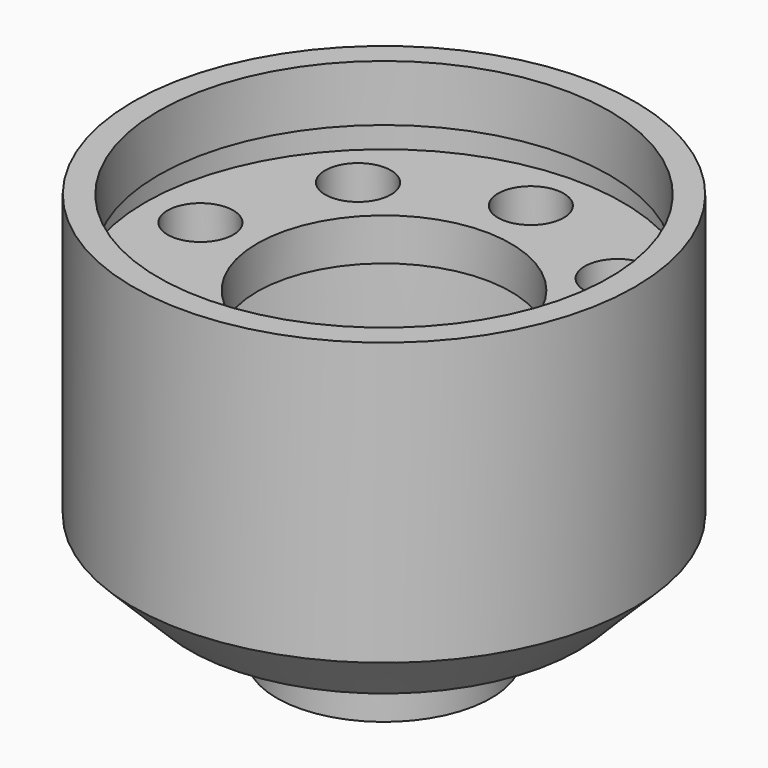
from build123d import *

# Parameters (mm, degrees)
F0_W     = 2.5722222222
F0_H     = 10.2888888889
F2_R     = 6
F3_DEPTH = 12.5


# Not quite as in the source:
# - ends of sketch curves that miss each other by under 0.0002 mm in the source are joined
# - a feature names something its author has since deleted; it is built from what else it names


with BuildPart() as f1:
    # F0 (on Front) → F1 (revolve)
    with BuildSketch(Plane.XZ):
        Polygon((-42.2873333333, 14.7902777778), (-43.4808444444, 14.7902777778), (-43.7277777778, 14.7902777778), (-43.7277777778, 25.0791666667), (-43.7277777778, 27.6513888889), (-43.7277777778, 37.9402777778), (-45.7855555556, 37.9402777778), (-45.7855555556, -13.5041666667), (-35.4966666667, -23.7930555556), (-23.15, -23.7930555556), (-19.5720388889, -23.7930555556), (-19.5488888889, -23.7930555556), (-19.5488888889, -36.6541666667), (-17.1001333333, -36.6541666667), (-17.1001333333, -35.0491), (-17.1307942222, -33.3098044889), (-16.0422915111, -33.2906054222), (-16.0422915111, -33.2845967111), (-16.0422915111, -33.278588), (-16.0422915111, -33.2725792889), (-16.0422915111, -33.2665705778), (-16.0422915111, -33.2605618667), (-16.0422915111, -33.2545531556), (-16.0422915111, -33.2485444444), (-16.0422915111, -33.2425357333), (-16.0422915111, -33.2365270222), (-16.0422915111, -33.2305183111), (-16.0422915111, -33.2245096), (-16.0422915111, -33.2185008889), (-16.0422915111, -33.2124921778), (-16.0422915111, -33.2064834667), (-16.0422915111, -33.2004747556), (-16.0422915111, -33.1944660444), (-16.0422915111, -33.1884573333), (-16.0422915111, -33.1824486222), (-16.0422915111, -33.1764604889), (-16.0422915111, -33.1704517778), (-16.0422915111, -33.1644430667), (-16.0422915111, -33.1584343556), (-16.0422915111, -33.1524256444), (-16.0422915111, -33.1464169333), (-16.0426824889, -33.1284731111), (-16.0438554222, -33.1105292889), (-16.0458103111, -33.0926677778), (-16.0485471556, -33.074868), (-16.0520659556, -33.0572534222), (-16.0563255556, -33.0398240444), (-16.0613465333, -33.0226004444), (-16.0671288889, -33.0056032), (-16.0736314667, -32.9888734667), (-16.0808748444, -32.9724112444), (-16.0888384444, -32.9562782667), (-16.0975016889, -32.9405156889), (-16.1068028444, -32.9251646667), (-16.1167830667, -32.9102663556), (-16.1273806222, -32.8958207556), (-16.1385955111, -32.8818484444), (-16.1504071556, -32.86837), (-16.1628361333, -32.855406), (-16.1758001333, -32.8429770222), (-16.1893403111, -32.8311036444), (-16.2033537778, -32.8198681778), (-16.2178405333, -32.8092500444), (-16.2327388444, -32.7992904), (-16.2480692889, -32.7899892444), (-16.2772074222, -32.7731772), (-16.3063455556, -32.7563445778), (-16.3354836889, -32.7395119556), (-16.3646218222, -32.7226999111), (-16.3937599556, -32.7058672889), (-16.4229186667, -32.6890552444), (-16.4520568, -32.6722226222), (-16.4811949333, -32.65539), (-16.5103330667, -32.6385779556), (-16.5394712, -32.6217453333), (-16.5686093333, -32.6049127111), (-16.5977474667, -32.5881006667), (-16.6268856, -32.5712680444), (-16.6560443111, -32.554456), (-16.6851824444, -32.5376233778), (-16.7143205778, -32.5207907556), (-16.7434587111, -32.5039787111), (-16.7725968444, -32.4871460889), (-16.8017349778, -32.4703340444), (-16.8308731111, -32.4535014222), (-16.8600318222, -32.4366688), (-16.8891699556, -32.4198567556), (-16.9183080889, -32.4030241333), (-16.9474462222, -32.3862120889), (-16.9625708889, -32.3770344), (-16.977284, -32.3672188), (-16.9915444, -32.3568064444), (-17.0053315111, -32.3457973333), (-17.0186453333, -32.3341914667), (-17.0314447111, -32.32203), (-17.0437296444, -32.3093129333), (-17.0554795556, -32.2960608444), (-17.0666327111, -32.2823354667), (-17.0771685333, -32.2681573778), (-17.0870870222, -32.2535471556), (-17.0963676, -32.2385253778), (-17.1049896889, -32.2231332), (-17.1129532889, -32.2073500444), (-17.1202584, -32.1912376444), (-17.1268432889, -32.1748165778), (-17.1327285333, -32.1581485778), (-17.1378729778, -32.1412748), (-17.1422766222, -32.1242158222), (-17.1459600444, -32.1069716444), (-17.1489026667, -32.089604), (-17.1511044889, -32.0720923111), (-17.1525449333, -32.0544777333), (-17.1532445778, -32.0368014222), (-17.1690071556, -31.1425529333), (-17.1689248444, -31.1242387111), (-17.16804, -31.1059862222), (-17.1663320444, -31.0878160444), (-17.1638215556, -31.0697281778), (-17.1605291111, -31.0517843556), (-17.1564341333, -31.0339845778), (-17.1515366222, -31.0163494222), (-17.1458571556, -30.9989406222), (-17.1394368889, -30.9818199111), (-17.1322552444, -30.9650284444), (-17.1243328, -30.9485662222), (-17.1157107111, -30.9324949778), (-17.1063684, -30.9167941333), (-17.0963264444, -30.9015254222), (-17.085626, -30.8867094222), (-17.0742464889, -30.8723461333), (-17.0622702222, -30.8585590222), (-17.0497177778, -30.8453069333), (-17.0365891556, -30.8326516), (-17.0229255111, -30.8205724444), (-17.0087268444, -30.8091312), (-16.9940343111, -30.7983072889), (-16.9788684889, -30.7881418667), (-16.9632293778, -30.7786349333), (-16.9359432444, -30.7628929333), (-16.9086571111, -30.7471303556), (-16.8813915556, -30.7313883556), (-16.8541054222, -30.7156463556), (-16.8268192889, -30.6998837778), (-16.7995537333, -30.6841417778), (-16.7722676, -30.6683997778), (-16.7449814667, -30.6526372), (-16.7177159111, -30.6368952), (-16.6904297778, -30.6211532), (-16.6631436444, -30.6053906222), (-16.6358780889, -30.5896486222), (-16.6085919556, -30.5738860444), (-16.5813058222, -30.5581440444), (-16.5540402667, -30.5424020444), (-16.5267541333, -30.5266394667), (-16.4994885778, -30.5108974667), (-16.4722024444, -30.4951554667), (-16.4449163111, -30.4793928889), (-16.4176507556, -30.4636508889), (-16.3903646222, -30.4478883111), (-16.3630784889, -30.4321463111), (-16.3358129333, -30.4164043111), (-16.3085268, -30.4006417333), (-16.2931757778, -30.3913405778), (-16.2782363111, -30.3813603556), (-16.2637289778, -30.3707216444), (-16.2497155111, -30.3594656), (-16.2361959111, -30.3476128), (-16.2232319111, -30.3351838222), (-16.2108235111, -30.3222198222), (-16.1989912889, -30.3087208), (-16.1877558222, -30.2947279111), (-16.1771376889, -30.2802205778), (-16.1671368889, -30.2652605333), (-16.1578151556, -30.2498889333), (-16.1491930667, -30.2341469333), (-16.1412706222, -30.2180756889), (-16.1340478222, -30.2016546222), (-16.1275452444, -30.1849660444), (-16.1217834667, -30.1679893778), (-16.1167624889, -30.1507452), (-16.1125028889, -30.1332952444), (-16.1089840889, -30.1156395111), (-16.1062678222, -30.0978808889), (-16.1043129333, -30.0800399556), (-16.10314, -30.0621578667), (-16.1027490222, -30.0442346222), (-16.1027490222, -30.0374028), (-16.1027490222, -30.0305915556), (-16.1027490222, -30.0237803111), (-16.1027490222, -30.0169484889), (-16.1027490222, -30.0101372444), (-16.1027490222, -30.003326), (-16.1027490222, -29.9964941778), (-16.1027490222, -29.9896829333), (-16.1027490222, -29.9828511111), (-16.1027490222, -29.9760398667), (-16.1027490222, -29.9692286222), (-16.1027490222, -29.9623968), (-16.1027490222, -29.9555855556), (-16.1027490222, -29.9487743111), (-16.1027490222, -29.9419424889), (-16.1027490222, -29.9351312444), (-16.1027490222, -29.9282994222), (-16.1027490222, -29.9214881778), (-16.1027490222, -29.9146769333), (-16.1027490222, -29.9078451111), (-16.1027490222, -29.9010338667), (-16.1027490222, -29.8942226222), (-16.1027490222, -29.8873908), (-16.1027490222, -29.8805795556), (-16.1027490222, -29.8737477333), (-16.1027490222, -29.8669364889), (-16.1027490222, -29.8601252444), (-16.1027490222, -29.8532934222), (-16.1027490222, -29.8464821778), (-16.1027490222, -29.8396709333), (-16.1027490222, -29.8328391111), (-16.1027490222, -29.8260278667), (-16.1027490222, -29.8191960444), (-16.1027490222, -29.8123848), (-16.1027490222, -29.8055735556), (-16.1027490222, -29.7987417333), (-16.1027490222, -29.7919304889), (-16.1027490222, -29.7851192444), (-16.1027490222, -29.7782874222), (-16.1027490222, -29.7714761778), (-16.1027490222, -29.7646443556), (-16.1027490222, -29.7578331111), (-16.1027490222, -29.7510218667), (-16.1027490222, -29.7441900444), (-16.1027490222, -29.7373788), (-16.1027490222, -29.7305675556), (-16.1027490222, -29.7237357333), (-16.1027490222, -29.7169244889), (-16.10314, -29.6989806667), (-16.1043129333, -29.6810574222), (-16.1062678222, -29.6631753333), (-16.1090046667, -29.6453755556), (-16.1125234667, -29.6277609778), (-16.1167830667, -29.6103316), (-16.1218246222, -29.593108), (-16.1275864, -29.5761107556), (-16.1340889778, -29.5593810222), (-16.1413323556, -29.5429188), (-16.1492959556, -29.5267858222), (-16.1579592, -29.5110232444), (-16.1672603556, -29.4956928), (-16.1772405778, -29.4807739111), (-16.1878381333, -29.4663283111), (-16.1990530222, -29.452356), (-16.2108852444, -29.4388775556), (-16.2232936444, -29.4259135556), (-16.2362576444, -29.4134845778), (-16.2497978222, -29.4016112), (-16.2638112889, -29.3903757333), (-16.2782980444, -29.3797576), (-16.2931963556, -29.3697979556), (-16.3085268, -29.3604968), (-16.3376649333, -29.3436847556), (-16.3668030667, -29.3268521333), (-16.3959412, -29.3100195111), (-16.4250999111, -29.2932074667), (-16.4542380444, -29.2763748444), (-16.4833761778, -29.2595628), (-16.5125143111, -29.2427301778), (-16.5416524444, -29.2258975556), (-16.5707905778, -29.2090855111), (-16.5999287111, -29.1922528889), (-16.6290874222, -29.1754202667), (-16.6582255556, -29.1586082222), (-16.6873636889, -29.1417756), (-16.7165018222, -29.1249635556), (-16.7456399556, -29.1081309333), (-16.7747780889, -29.0912983111), (-16.8039368, -29.0744862667), (-16.8330749333, -29.0576536444), (-16.8622130667, -29.0408416), (-16.8913512, -29.0240089778), (-16.9204893333, -29.0071763556), (-16.9496274667, -28.9903643111), (-16.9787656, -28.9735316889), (-17.0079243111, -28.9566990667), (-17.0230489778, -28.9475419556), (-17.0377415111, -28.9377263556), (-17.0520019111, -28.927314), (-17.0658096, -28.9163048889), (-17.0791028444, -28.9046990222), (-17.0919228, -28.8925375556), (-17.1042077333, -28.8798204889), (-17.1159576444, -28.8665684), (-17.1270902222, -28.8528430222), (-17.1376260444, -28.8386649333), (-17.1475445333, -28.8240547111), (-17.1568251111, -28.8090329333), (-17.1654677778, -28.7936407556), (-17.1734313778, -28.7778576), (-17.1807364889, -28.7617246222), (-17.1873213778, -28.7453241333), (-17.1931860444, -28.7286561333), (-17.1983304889, -28.7117823556), (-17.2027547111, -28.6947233778), (-17.2064381333, -28.6774792), (-17.2093807556, -28.6601115556), (-17.2115825778, -28.6425998667), (-17.2130230222, -28.6249852889), (-17.2137226667, -28.6073089778), (-17.2441777778, -26.8797222222), (-17.3573555556, -26.8797222222), (-17.3573555556, -22.5583888889), (-17.8325787556, -21.7352777778), (-34.6443145333, -21.7352777778), (-42.0330537333, -14.346518), align=None)
        with Locations((-42.4416666667, 32.7958333333)):
            Rectangle(F0_W, F0_H)
        Polygon((-38.4037510667, 22.5069444444), (-41.1555555556, 22.5069444444), (-43.5481955111, 22.5069444444), (-43.4808444444, 14.7902777778), (-42.2873333333, 14.7902777778), (-41.4230666667, 14.7902777778), (-41.37368, 20.4491666667), (-38.4216948889, 20.4491666667), align=None)
        Polygon((-33.4388888889, 22.5069444444), (-38.4037510667, 22.5069444444), (-38.4216948889, 20.4491666667), (-23.15, 20.4491666667), (-23.15, 22.5069444444), align=None)
        Polygon((-23.15, 20.4491666667), (-38.4216948889, 20.4491666667), (-41.37368, 20.4491666667), (-41.4230666667, 14.7902777778), (-23.15, 14.7902777778), align=None)
    revolve(axis=Axis((0, 0, -1.0518405444), (0, 0, -1)))

    # F2 (on face) → F3 (cut)
    with BuildSketch(Plane.XY.offset(22.5069444444)):
        with Locations((0, 33.5)):
            Circle(F2_R)
        with Locations((23.6880771697, 23.6880771697)):
            Circle(F2_R)
        with Locations((33.5, 0)):
            Circle(F2_R)
        with Locations((23.6880771697, -23.6880771697)):
            Circle(F2_R)
        with Locations((0, -33.5)):
            Circle(F2_R)
        with Locations((-23.6880771697, -23.6880771697)):
            Circle(F2_R)
        with Locations((-33.5, 0)):
            Circle(F2_R)
        with Locations((-23.6880771697, 23.6880771697)):
            Circle(F2_R)
    extrude(amount=-F3_DEPTH, mode=Mode.SUBTRACT)


solid = f1.part
